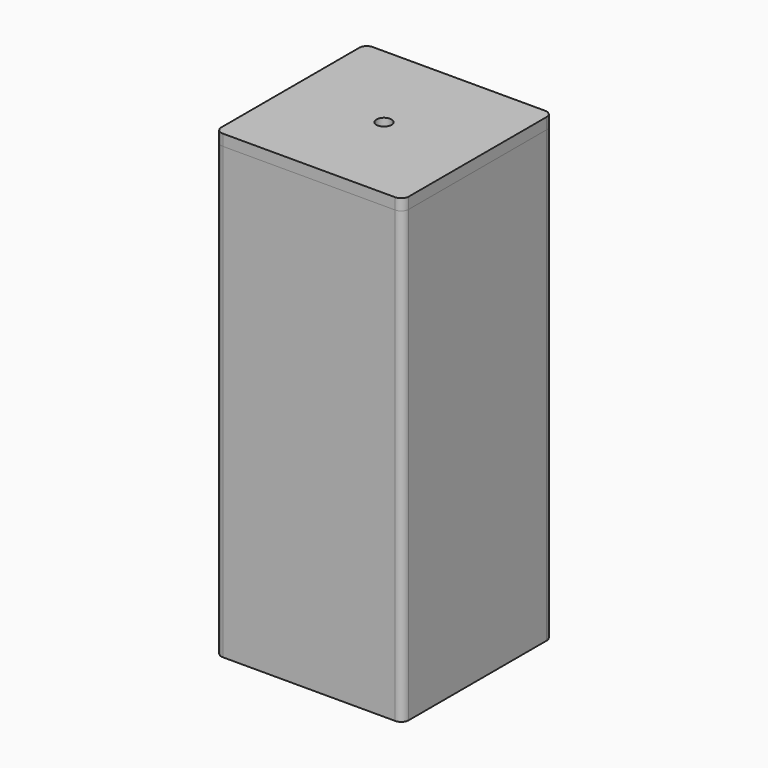
from build123d import *

# Parameters (mm, degrees)
F0_W          = 50
F0_H          = 50
F0_R          = 12
F1_DEPTH      = 120
F0_R_2        = 2
F2_DEPTH      = 3
F3_SIZE       = 11
F4_W          = 50
F4_H          = 50
F4_R          = 2
F5_DEPTH      = 3
F5_DEPTH_BACK = 11
F7_R          = 10
F8_DEPTH      = 11
F9_R          = 2
F9_2_R        = 2


# Not quite as in the source:
# - a feature names something its author has since deleted; it is built from what else it names


with BuildPart() as f1:
    # F0 (on Top) → F1 (new body)
    with BuildSketch(Plane.XY):
        Rectangle(F0_W, F0_H)
        Circle(F0_R, mode=Mode.SUBTRACT)
    extrude(amount=F1_DEPTH)

    # F0 (on Top) → F2 (join)
    with BuildSketch(Plane.XY):
        Circle(F0_R)
        Circle(F0_R_2, mode=Mode.SUBTRACT)
    extrude(amount=F2_DEPTH)

    # F3
    f3_edges = [f1.edges().sort_by_distance(p)[0] for p in [
        (-12, 0, 120),
    ]]
    chamfer(f3_edges, length=F3_SIZE)


with BuildPart() as f5:
    # F4 (on face) → F5 (new body, two sides)
    with BuildSketch(Plane.XY.offset(120)) as f5_sk:
        Rectangle(F4_W, F4_H)
        Circle(F4_R, mode=Mode.SUBTRACT)
    extrude(amount=F5_DEPTH)
    extrude(f5_sk.sketch, amount=-F5_DEPTH_BACK)

    # F6: cut F1
    add(f1.part, mode=Mode.SUBTRACT)

    # F7 (on face) → F8 (cut, through all)
    with BuildSketch(Plane(origin=(0, 0, 109), x_dir=(1, 0, 0), z_dir=(0, 0, -1))):
        Circle(F7_R)
    extrude(amount=-F8_DEPTH, mode=Mode.SUBTRACT)

    # F9#2
    f9_2_edges = [f5.edges().sort_by_distance(p)[0] for p in [
        (25, -25, 121.5),
        (25, 25, 121.5),
        (-25, 25, 121.5),
        (-25, -25, 121.5),
    ]]
    fillet(f9_2_edges, radius=F9_2_R)


with BuildPart() as f1_1:
    add(f1.part)

    # F9
    f9_edges = [f1_1.edges().sort_by_distance(p)[0] for p in [
        (25, -25, 60),
        (25, 25, 60),
        (-25, 25, 60),
        (-25, -25, 60),
    ]]
    fillet(f9_edges, radius=F9_R)


solid = Compound([f5.part, f1_1.part])
